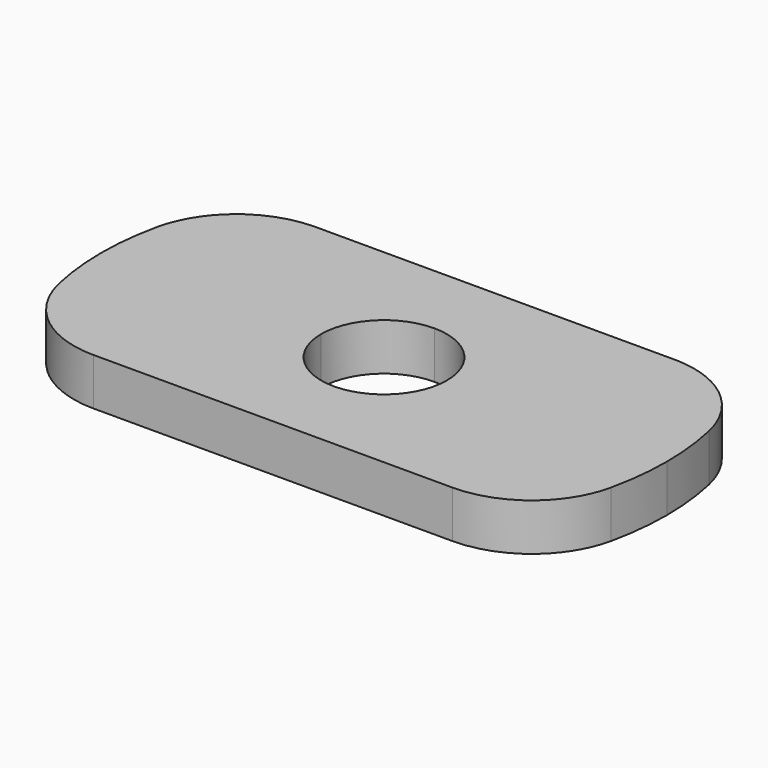
from build123d import *

# Parameters (mm, degrees)
F1_DEPTH = 4.7625
F2_R     = 10


# Not quite as in the source:
# - a feature names something its author has since deleted; it is built from what else it names


with BuildPart() as f1:
    # F0 (on Top) → F1 (new body)
    with BuildSketch(Plane.XY):
        with BuildLine():
            ThreePointArc((-6.35, 0), (-4.4901280605, 4.4901280605), (0, 6.35))
            Line((0, 6.35), (-12.4931629071, 6.35))
            ThreePointArc((-12.4931629071, 6.35), (-13.6287381062, 3.2648303256), (-14.0143362106, 0))
            Line((-14.0143362106, 0), (-6.35, 0))
        make_face()
        with BuildLine():
            ThreePointArc((0, 6.35), (4.4901280605, 4.4901280605), (6.35, 0))
            Line((6.35, 0), (14.0143362106, 0))
            ThreePointArc((14.0143362106, 0), (13.6287381062, 3.2648303256), (12.4931629071, 6.35))
            Line((12.4931629071, 6.35), (0, 6.35))
        make_face()
        with BuildLine():
            Line((12.4931629071, -6.35), (0, -6.35))
            Line((0, -6.35), (0, -14.0143362106))
            ThreePointArc((0, -14.0143362106), (7.3283894713, -11.9455567966), (12.4931629071, -6.35))
        make_face()
        with BuildLine():
            Line((0, -14.0143362106), (0, -6.35))
            Line((0, -6.35), (-12.4931629071, -6.35))
            ThreePointArc((-12.4931629071, -6.35), (-7.3283894713, -11.9455567966), (0, -14.0143362106))
        make_face()
        with BuildLine():
            Line((-12.4931629071, -6.35), (0, -6.35))
            ThreePointArc((0, -6.35), (-4.4901280605, -4.4901280605), (-6.35, 0))
            Line((-6.35, 0), (-14.0143362106, 0))
            ThreePointArc((-14.0143362106, 0), (-13.6287381062, -3.2648303256), (-12.4931629071, -6.35))
        make_face()
        with BuildLine():
            Line((-27.86051193, -6.35), (-12.4931629071, -6.35))
            ThreePointArc((-12.4931629071, -6.35), (-13.6287381062, -3.2648303256), (-14.0143362106, 0))
            Line((-14.0143362106, 0), (-28.575, 0))
            ThreePointArc((-28.575, 0), (-28.395816183, -3.1950349451), (-27.86051193, -6.35))
        make_face()
        with BuildLine():
            ThreePointArc((12.4931629071, 6.35), (13.6287381062, 3.2648303256), (14.0143362106, 0))
            Line((14.0143362106, 0), (28.575, 0))
            ThreePointArc((28.575, 0), (28.395816183, 3.1950349451), (27.86051193, 6.35))
            Line((27.86051193, 6.35), (12.4931629071, 6.35))
        make_face()
        with BuildLine():
            Line((0, 14.0143362106), (0, 6.35))
            Line((0, 6.35), (12.4931629071, 6.35))
            ThreePointArc((12.4931629071, 6.35), (7.3283894713, 11.9455567966), (0, 14.0143362106))
        make_face()
        with BuildLine():
            Line((-12.4931629071, 6.35), (0, 6.35))
            Line((0, 6.35), (0, 14.0143362106))
            ThreePointArc((0, 14.0143362106), (-7.3283894713, 11.9455567966), (-12.4931629071, 6.35))
        make_face()
        with BuildLine():
            Line((-24.9023895556, -14.0143362106), (0, -14.0143362106))
            ThreePointArc((0, -14.0143362106), (-7.3283894713, -11.9455567966), (-12.4931629071, -6.35))
            Line((-12.4931629071, -6.35), (-27.86051193, -6.35))
            ThreePointArc((-27.86051193, -6.35), (-26.6583280736, -10.2890315054), (-24.9023895556, -14.0143362106))
        make_face()
        with BuildLine():
            Line((24.9023895556, 14.0143362106), (0, 14.0143362106))
            ThreePointArc((0, 14.0143362106), (7.3283894713, 11.9455567966), (12.4931629071, 6.35))
            Line((12.4931629071, 6.35), (27.86051193, 6.35))
            ThreePointArc((27.86051193, 6.35), (26.6583280736, 10.2890315054), (24.9023895556, 14.0143362106))
        make_face()
        with BuildLine():
            Line((14.0143362106, 0), (6.35, 0))
            ThreePointArc((6.35, 0), (4.4901280605, -4.4901280605), (0, -6.35))
            Line((0, -6.35), (12.4931629071, -6.35))
            ThreePointArc((12.4931629071, -6.35), (13.6287381062, -3.2648303256), (14.0143362106, 0))
        make_face()
        with BuildLine():
            ThreePointArc((-14.0143362106, 0), (-13.6287381062, 3.2648303256), (-12.4931629071, 6.35))
            Line((-12.4931629071, 6.35), (-27.86051193, 6.35))
            ThreePointArc((-27.86051193, 6.35), (-28.395816183, 3.1950349451), (-28.575, 0))
            Line((-28.575, 0), (-14.0143362106, 0))
        make_face()
        with BuildLine():
            ThreePointArc((-12.4931629071, 6.35), (-7.3283894713, 11.9455567966), (0, 14.0143362106))
            Line((0, 14.0143362106), (-24.9023895556, 14.0143362106))
            ThreePointArc((-24.9023895556, 14.0143362106), (-26.6583280736, 10.2890315054), (-27.86051193, 6.35))
            Line((-27.86051193, 6.35), (-12.4931629071, 6.35))
        make_face()
        with BuildLine():
            Line((28.575, 0), (14.0143362106, 0))
            ThreePointArc((14.0143362106, 0), (13.6287381062, -3.2648303256), (12.4931629071, -6.35))
            Line((12.4931629071, -6.35), (27.86051193, -6.35))
            ThreePointArc((27.86051193, -6.35), (28.395816183, -3.1950349451), (28.575, 0))
        make_face()
        with BuildLine():
            ThreePointArc((12.4931629071, -6.35), (7.3283894713, -11.9455567966), (0, -14.0143362106))
            Line((0, -14.0143362106), (24.9023895556, -14.0143362106))
            ThreePointArc((24.9023895556, -14.0143362106), (26.6583280736, -10.2890315054), (27.86051193, -6.35))
            Line((27.86051193, -6.35), (12.4931629071, -6.35))
        make_face()
    extrude(amount=F1_DEPTH)

    # F2
    f2_edges = [f1.edges().sort_by_distance(p)[0] for p in [
        (24.90239, 14.014336, 2.38125),
        (-24.90239, 14.014336, 2.38125),
        (24.90239, -14.014336, 2.38125),
        (-24.90239, -14.014336, 2.38125),
    ]]
    fillet(f2_edges, radius=F2_R)


solid = f1.part
